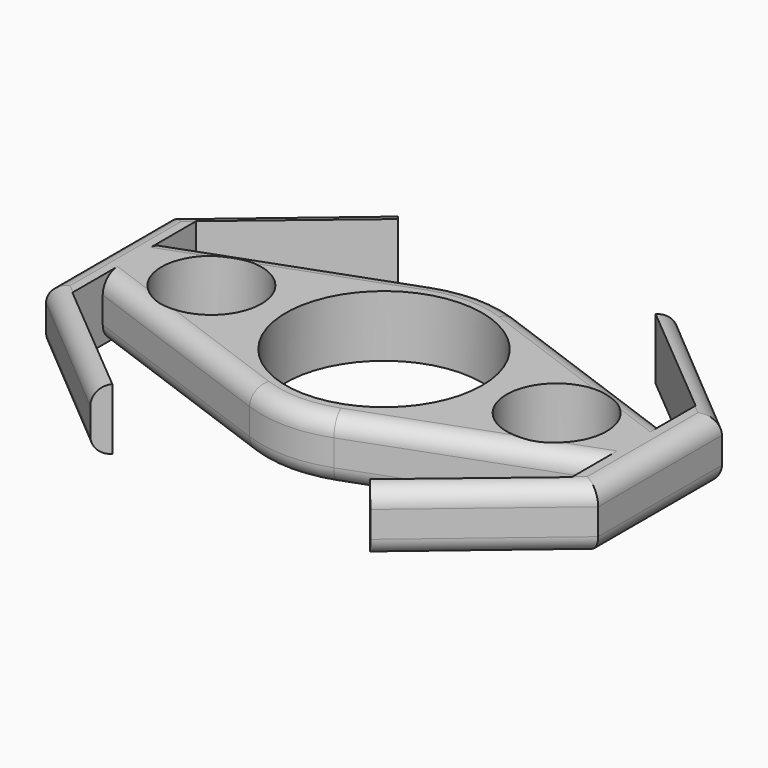
from build123d import *

# Parameters (mm, degrees)
F0_R         = 5.7
F0_R_2       = 11.2
F1_DEPTH     = 7
F2_T1_DEPTH  = 30.3000361162
F2_T3_DEPTH  = 27.6438093403
F2_T5_DEPTH  = 30.3000361162
F2_T7_DEPTH  = 30.3000361162
F2_T9_DEPTH  = 30.3000361162
F2_T14_DEPTH = 30.2088556234
F2_T19_DEPTH = 30.2088556234
F2_T24_DEPTH = 30.2088556234
F2_T29_DEPTH = 30.2088556234
F2_T34_DEPTH = 30.2088556234
F2_T37_ANGLE = 40.1571894023
F2_T39_ANGLE = 40.1571894023
F2_T43_DEPTH = 30.2088556234
F2_T48_DEPTH = 30.2088556234
F2_T51_ANGLE = 40.1571894023
F2_T53_ANGLE = 40.1571894023
F2_T57_DEPTH = 30.2088556234


# Not quite as in the source:
# - a fillet or chamfer that OpenCascade refuses, or shapes differently, is made with other operations: its cross-section is extruded or revolved along the edge and cut away or added


with BuildPart() as f1:
    # F0 (on Top) → F1 (new body)
    with BuildSketch(Plane.XY):
        with BuildLine():
            Line((-28.483049944, -4.4946932848), (-4.8063236428, -13.1491160555))
            ThreePointArc((-4.8063236428, -13.1491160555), (0, -14), (4.8063236428, -13.1491160555))
            Line((4.8063236428, -13.1491160555), (28.483049944, -4.4946932848))
            Line((28.483049944, -4.4946932848), (28.483049944, -8.8219046702))
            Line((28.483049944, -8.8219046702), (14.6836369881, -20.3794217941))
            Line((14.6836369881, -20.3794217941), (15.9678055574, -21.9126899004))
            Line((15.9678055574, -21.9126899004), (31.483049944, -8.8219046702))
            Line((31.483049944, -8.8219046702), (31.483049944, 8.8219046702))
            Line((31.483049944, 8.8219046702), (15.9678055574, 21.9126899004))
            Line((15.9678055574, 21.9126899004), (14.6836369881, 20.3794217941))
            Line((14.6836369881, 20.3794217941), (28.483049944, 8.8219046702))
            Line((28.483049944, 8.8219046702), (28.483049944, 4.4946932848))
            Line((28.483049944, 4.4946932848), (4.8063236428, 13.1491160555))
            ThreePointArc((4.8063236428, 13.1491160555), (0, 14), (-4.8063236428, 13.1491160555))
            Line((-4.8063236428, 13.1491160555), (-28.483049944, 4.4946932848))
            Line((-28.483049944, 4.4946932848), (-28.483049944, 8.8219046702))
            Line((-28.483049944, 8.8219046702), (-14.6836369881, 20.3794217941))
            Line((-14.6836369881, 20.3794217941), (-15.9678055574, 21.9126899004))
            Line((-15.9678055574, 21.9126899004), (-31.483049944, 8.8219046702))
            Line((-31.483049944, 8.8219046702), (-31.483049944, -8.8219046702))
            Line((-31.483049944, -8.8219046702), (-15.9678055574, -21.9126899004))
            Line((-15.9678055574, -21.9126899004), (-14.6836369881, -20.3794217941))
            Line((-14.6836369881, -20.3794217941), (-28.483049944, -8.8219046702))
            Line((-28.483049944, -8.8219046702), (-28.483049944, -4.4946932848))
        make_face()
        with Locations((-19.682828337, 0)):
            Circle(F0_R, mode=Mode.SUBTRACT)
        Circle(F0_R_2, mode=Mode.SUBTRACT)
        with Locations((19.682828337, 0)):
            Circle(F0_R, mode=Mode.SUBTRACT)
    extrude(amount=F1_DEPTH)

    # F2: fillet of radius 2 on 24 edges, made by hand

    # F2_s2 → F2_t1 (cut)
    with BuildSketch(Plane(origin=(17.8642381106, -15.0727180688, 0), x_dir=(0, 0, 1), z_dir=(-0.7642963933, 0.6448651202, 0))):
        with BuildLine():
            ThreePointArc((5, 27.0448707076), (6.4142135624, 26.4590842699), (7, 25.0448707076))
            Line((7, 25.0448707076), (7, 27.0448707076))
            Line((7, 27.0448707076), (5, 27.0448707076))
        make_face()
        with BuildLine():
            ThreePointArc((2, 27.0448707076), (0.5857864376, 26.4590842699), (0, 25.0448707076))
            Line((0, 25.0448707076), (0, 27.0448707076))
            Line((0, 27.0448707076), (2, 27.0448707076))
        make_face()
    extrude(amount=F2_T1_DEPTH, mode=Mode.SUBTRACT)

    # F2_s4 → F2_t3 (cut)
    with BuildSketch(Plane.XZ.offset(-13.8219046702)):
        with BuildLine():
            ThreePointArc((31.483049944, 5), (30.8972635064, 6.4142135624), (29.483049944, 7))
            Line((29.483049944, 7), (31.483049944, 7))
            Line((31.483049944, 7), (31.483049944, 5))
        make_face()
        with BuildLine():
            ThreePointArc((31.483049944, 2), (30.8972635064, 0.5857864376), (29.483049944, 0))
            Line((29.483049944, 0), (31.483049944, 0))
            Line((31.483049944, 0), (31.483049944, 2))
        make_face()
        with BuildLine():
            ThreePointArc((-31.483049944, 5), (-30.8972635064, 6.4142135624), (-29.483049944, 7))
            Line((-29.483049944, 7), (-31.483049944, 7))
            Line((-31.483049944, 7), (-31.483049944, 5))
        make_face()
        with BuildLine():
            ThreePointArc((-31.483049944, 2), (-30.8972635064, 0.5857864376), (-29.483049944, 0))
            Line((-29.483049944, 0), (-31.483049944, 0))
            Line((-31.483049944, 0), (-31.483049944, 2))
        make_face()
    extrude(amount=F2_T3_DEPTH, mode=Mode.SUBTRACT)

    # F2_s6 → F2_t5 (cut)
    with BuildSketch(Plane(origin=(-5.2939702086, -4.4667183635, 0), x_dir=(0, 0, 1), z_dir=(0.7642963933, 0.6448651202, 0))):
        with BuildLine():
            ThreePointArc((5, 27.0448707076), (6.4142135624, 26.4590842699), (7, 25.0448707076))
            Line((7, 25.0448707076), (7, 27.0448707076))
            Line((7, 27.0448707076), (5, 27.0448707076))
        make_face()
        with BuildLine():
            ThreePointArc((2, 27.0448707076), (0.5857864376, 26.4590842699), (0, 25.0448707076))
            Line((0, 25.0448707076), (0, 27.0448707076))
            Line((0, 27.0448707076), (2, 27.0448707076))
        make_face()
    extrude(amount=F2_T5_DEPTH, mode=Mode.SUBTRACT)

    # F2_s8 → F2_t7 (cut)
    with BuildSketch(Plane(origin=(5.2939702086, 4.4667183635, 0), x_dir=(0, 0, 1), z_dir=(-0.7642963933, -0.6448651202, 0))):
        with BuildLine():
            ThreePointArc((5, 27.0448707076), (6.4142135624, 26.4590842699), (7, 25.0448707076))
            Line((7, 25.0448707076), (7, 27.0448707076))
            Line((7, 27.0448707076), (5, 27.0448707076))
        make_face()
        with BuildLine():
            ThreePointArc((2, 27.0448707076), (0.5857864376, 26.4590842699), (0, 25.0448707076))
            Line((0, 25.0448707076), (0, 27.0448707076))
            Line((0, 27.0448707076), (2, 27.0448707076))
        make_face()
    extrude(amount=F2_T7_DEPTH, mode=Mode.SUBTRACT)

    # F2_s10 → F2_t9 (cut)
    with BuildSketch(Plane(origin=(-17.8642381106, 15.0727180688, 0), x_dir=(0, 0, 1), z_dir=(0.7642963933, -0.6448651202, 0))):
        with BuildLine():
            ThreePointArc((5, 27.0448707076), (6.4142135624, 26.4590842699), (7, 25.0448707076))
            Line((7, 25.0448707076), (7, 27.0448707076))
            Line((7, 27.0448707076), (5, 27.0448707076))
        make_face()
        with BuildLine():
            ThreePointArc((2, 27.0448707076), (0.5857864376, 26.4590842699), (0, 25.0448707076))
            Line((0, 25.0448707076), (0, 27.0448707076))
            Line((0, 27.0448707076), (2, 27.0448707076))
        make_face()
    extrude(amount=F2_T9_DEPTH, mode=Mode.SUBTRACT)


with BuildPart() as f2_tool12:
    # F2_s13 → F2_t14 (new body)
    with BuildSketch(Plane(origin=(-28.3728391782, 10.3709669288, 0), x_dir=(0, 0, 1), z_dir=(0.9392225754, -0.3433088316, 0))):
        with BuildLine():
            ThreePointArc((5, 14), (6.4142135624, 13.4142135624), (7, 12))
            Line((7, 12), (7, 14))
            Line((7, 14), (5, 14))
        make_face()
    extrude(amount=F2_T14_DEPTH)

    split(bisect_by=Plane.YZ.offset(-28.483049944), keep=Keep.TOP)


with BuildPart() as f1_1:
    add(f1.part)

    # F2_t11: cut F2_tool12
    add(f2_tool12.part, mode=Mode.SUBTRACT)


with BuildPart() as f2_tool17:
    # F2_s18 → F2_t19 (new body)
    with BuildSketch(Plane(origin=(0, 0, 0), x_dir=(0, 0, 1), z_dir=(-0.9392225754, -0.3433088316, 0))):
        with BuildLine():
            ThreePointArc((5, 14), (6.4142135624, 13.4142135624), (7, 12))
            Line((7, 12), (7, 14))
            Line((7, 14), (5, 14))
        make_face()
    extrude(amount=F2_T19_DEPTH)

    split(bisect_by=Plane.YZ.offset(-28.483049944), keep=Keep.TOP)


with BuildPart() as f1_2:
    add(f1_1.part)

    # F2_t16: cut F2_tool17
    add(f2_tool17.part, mode=Mode.SUBTRACT)


with BuildPart() as f2_tool22:
    # F2_s23 → F2_t24 (new body)
    with BuildSketch(Plane(origin=(0, 0, 0), x_dir=(0, 0, 1), z_dir=(0.9392225754, 0.3433088316, 0))):
        with BuildLine():
            ThreePointArc((2, 14), (0.5857864376, 13.4142135624), (0, 12))
            Line((0, 12), (0, 14))
            Line((0, 14), (2, 14))
        make_face()
    extrude(amount=F2_T24_DEPTH)

    split(bisect_by=Plane.YZ.offset(28.483049944), keep=Keep.BOTTOM)


with BuildPart() as f1_3:
    add(f1_2.part)

    # F2_t21: cut F2_tool22
    add(f2_tool22.part, mode=Mode.SUBTRACT)


with BuildPart() as f2_tool27:
    # F2_s28 → F2_t29 (new body)
    with BuildSketch(Plane(origin=(28.3728391782, -10.3709669288, 0), x_dir=(0, 0, 1), z_dir=(-0.9392225754, 0.3433088316, 0))):
        with BuildLine():
            ThreePointArc((2, 14), (0.5857864376, 13.4142135624), (0, 12))
            Line((0, 12), (0, 14))
            Line((0, 14), (2, 14))
        make_face()
    extrude(amount=F2_T29_DEPTH)

    split(bisect_by=Plane.YZ.offset(28.483049944), keep=Keep.BOTTOM)


with BuildPart() as f1_4:
    add(f1_3.part)

    # F2_t26: cut F2_tool27
    add(f2_tool27.part, mode=Mode.SUBTRACT)


with BuildPart() as f2_tool32:
    # F2_s33 → F2_t34 (new body)
    with BuildSketch(Plane(origin=(-28.3728391782, 10.3709669288, 0), x_dir=(0, 0, 1), z_dir=(0.9392225754, -0.3433088316, 0))):
        with BuildLine():
            ThreePointArc((2, 14), (0.5857864376, 13.4142135624), (0, 12))
            Line((0, 12), (0, 14))
            Line((0, 14), (2, 14))
        make_face()
    extrude(amount=F2_T34_DEPTH)

    split(bisect_by=Plane.YZ.offset(-28.483049944), keep=Keep.TOP)


with BuildPart() as f1_5:
    add(f1_4.part)

    # F2_t31: cut F2_tool32
    add(f2_tool32.part, mode=Mode.SUBTRACT)

    # F2_s36 → F2_t37 (revolve, cut)
    with BuildSketch(Plane(origin=(0, 0, 0), x_dir=(0, 0, 1), z_dir=(-0.9392225754, 0.3433088316, 0))):
        with BuildLine():
            ThreePointArc((2, -14), (0.5857864376, -13.4142135624), (0, -12))
            Line((0, -12), (0, -14))
            Line((0, -14), (2, -14))
        make_face()
    revolve(axis=Axis((0, 0, 0), (0, 0, 1)), revolution_arc=F2_T37_ANGLE, mode=Mode.SUBTRACT)

    # F2_s38 → F2_t39 (revolve, cut)
    with BuildSketch(Plane(origin=(0, 0, 0), x_dir=(0, 0, 1), z_dir=(-0.9392225754, 0.3433088316, 0))):
        with BuildLine():
            ThreePointArc((5, -14), (6.4142135624, -13.4142135624), (7, -12))
            Line((7, -12), (7, -14))
            Line((7, -14), (5, -14))
        make_face()
    revolve(axis=Axis((0, 0, 7), (0, 0, 1)), revolution_arc=F2_T39_ANGLE, mode=Mode.SUBTRACT)


with BuildPart() as f2_tool41:
    # F2_s42 → F2_t43 (new body)
    with BuildSketch(Plane(origin=(0, 0, 0), x_dir=(0, 0, 1), z_dir=(0.9392225754, 0.3433088316, 0))):
        with BuildLine():
            ThreePointArc((5, 14), (6.4142135624, 13.4142135624), (7, 12))
            Line((7, 12), (7, 14))
            Line((7, 14), (5, 14))
        make_face()
    extrude(amount=F2_T43_DEPTH)

    split(bisect_by=Plane.YZ.offset(28.483049944), keep=Keep.BOTTOM)


with BuildPart() as f1_6:
    add(f1_5.part)

    # F2_t40: cut F2_tool41
    add(f2_tool41.part, mode=Mode.SUBTRACT)


with BuildPart() as f2_tool46:
    # F2_s47 → F2_t48 (new body)
    with BuildSketch(Plane(origin=(28.3728391782, -10.3709669288, 0), x_dir=(0, 0, 1), z_dir=(-0.9392225754, 0.3433088316, 0))):
        with BuildLine():
            ThreePointArc((5, 14), (6.4142135624, 13.4142135624), (7, 12))
            Line((7, 12), (7, 14))
            Line((7, 14), (5, 14))
        make_face()
    extrude(amount=F2_T48_DEPTH)

    split(bisect_by=Plane.YZ.offset(28.483049944), keep=Keep.BOTTOM)


with BuildPart() as f1_7:
    add(f1_6.part)

    # F2_t45: cut F2_tool46
    add(f2_tool46.part, mode=Mode.SUBTRACT)

    # F2_s50 → F2_t51 (revolve, cut)
    with BuildSketch(Plane(origin=(0, 0, 0), x_dir=(0, 0, 1), z_dir=(0.9392225754, -0.3433088316, 0))):
        with BuildLine():
            ThreePointArc((2, -14), (0.5857864376, -13.4142135624), (0, -12))
            Line((0, -12), (0, -14))
            Line((0, -14), (2, -14))
        make_face()
    revolve(axis=Axis((0, 0, 0), (0, 0, 1)), revolution_arc=F2_T51_ANGLE, mode=Mode.SUBTRACT)

    # F2_s52 → F2_t53 (revolve, cut)
    with BuildSketch(Plane(origin=(0, 0, 0), x_dir=(0, 0, 1), z_dir=(0.9392225754, -0.3433088316, 0))):
        with BuildLine():
            ThreePointArc((5, -14), (6.4142135624, -13.4142135624), (7, -12))
            Line((7, -12), (7, -14))
            Line((7, -14), (5, -14))
        make_face()
    revolve(axis=Axis((0, 0, 7), (0, 0, 1)), revolution_arc=F2_T53_ANGLE, mode=Mode.SUBTRACT)


with BuildPart() as f2_tool55:
    # F2_s56 → F2_t57 (new body)
    with BuildSketch(Plane(origin=(0, 0, 0), x_dir=(0, 0, 1), z_dir=(-0.9392225754, -0.3433088316, 0))):
        with BuildLine():
            ThreePointArc((2, 14), (0.5857864376, 13.4142135624), (0, 12))
            Line((0, 12), (0, 14))
            Line((0, 14), (2, 14))
        make_face()
    extrude(amount=F2_T57_DEPTH)

    split(bisect_by=Plane.YZ.offset(-28.483049944), keep=Keep.TOP)


with BuildPart() as f1_8:
    add(f1_7.part)

    # F2_t54: cut F2_tool55
    add(f2_tool55.part, mode=Mode.SUBTRACT)


solid = f1_8.part
